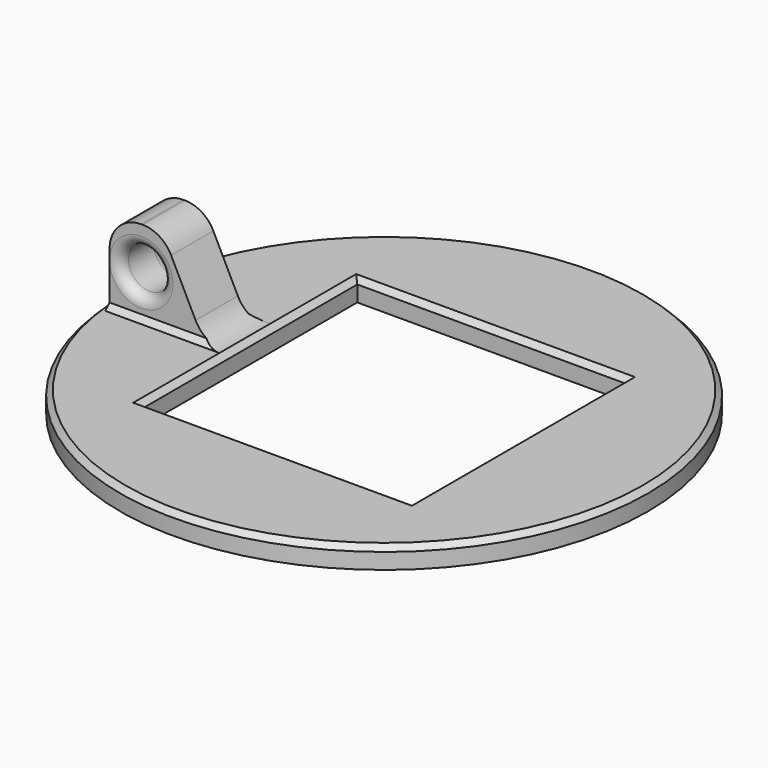
from build123d import *

# Parameters (mm, degrees)
F0_R          = 25
F0_W          = 25.4
F0_H          = 25.4
F1_DEPTH      = 2
F2_R          = 2
F3_DEPTH      = 2.5
F3_DEPTH_BACK = 2.5
F4_SIZE       = 0.5
F5_R          = 0.99999
F6_T4_DEPTH   = 5
F6_T9_DEPTH   = 5.1486606532
F6_T15_DEPTH  = 5.1486606532
F6_T18_DEPTH  = 20
F6_T20_DEPTH  = 14.2973213065


# Not quite as in the source:
# - a fillet or chamfer that OpenCascade refuses, or shapes differently, is made with other operations: its cross-section is extruded or revolved along the edge and cut away or added
# - a fillet or chamfer is up to 0.001 mm smaller than in the source, because OpenCascade refuses the exact size


with BuildPart() as f1:
    # F0 (on Top) → F1 (new body)
    with BuildSketch(Plane.XY):
        Circle(F0_R)
        Rectangle(F0_W, F0_H, mode=Mode.SUBTRACT)
    extrude(amount=F1_DEPTH)

    # F2 (on Front) → F3 (join, two sides)
    with BuildSketch(Plane.XZ) as f3_sk:
        Polygon((-24, 10), (-24, 1.4085747534), (-14.7320097312, 1.4085747534), (-19, 10), align=None)
        with Locations((-21, 6)):
            Circle(F2_R, mode=Mode.SUBTRACT)
    extrude(amount=F3_DEPTH)
    extrude(f3_sk.sketch, amount=-F3_DEPTH_BACK)

    # F4
    f4_edges = [f1.edges().sort_by_distance(p)[0] for p in [
        (0, 12.7, 2),
        (12.7, 0, 2),
        (0, -12.7, 2),
        (-12.7, 0, 2),
        (-25, 0, 2),
        (-19.512907, 2.5, 2),
        (-19.512907, -2.5, 2),
    ]]
    chamfer(f4_edges, length=F4_SIZE)

    # F5 (radius 1 in the source; OpenCascade refuses exactly that, so slightly less here)
    f5_edges = [f1.edges().sort_by_distance(p)[0] for p in [
        (-23, -2.5, 6),
        (-23, 2.5, 6),
    ]]
    fillet(f5_edges, radius=F5_R)

    # F6: fillet of radius 3 on 3 edges, made by hand


with BuildPart() as f6_tool2:
    # F6_s3 → F6_t4 (new body)
    with BuildSketch(Plane.XZ.offset(-2.5)):
        with BuildLine():
            ThreePointArc((-15.8530900959, 3.66529924), (-14.7468397832, 2.4500880133), (-13.1663497137, 2))
            Line((-13.1663497137, 2), (-15.025813975, 2))
            Line((-15.025813975, 2), (-15.8530900959, 3.66529924))
        make_face()
    extrude(amount=F6_T4_DEPTH)

    split(bisect_by=Plane(origin=(-5.6, 0, -5.6), x_dir=(0, 1, 0), z_dir=(-0.7071067812, 0, -0.7071067812)), keep=Keep.TOP)


with BuildPart() as f1_1:
    add(f1.part)

    # F6_t1: union F6_tool2
    add(f6_tool2.part)


with BuildPart() as f6_tool7:
    # F6_s8 → F6_t9 (new body)
    with BuildSketch(Plane.XZ.offset(-2.5)):
        with BuildLine():
            ThreePointArc((-15.8530900959, 3.66529924), (-14.7468397832, 2.4500880133), (-13.1663497137, 2))
            Line((-13.1663497137, 2), (-15.025813975, 2))
            Line((-15.025813975, 2), (-15.8530900959, 3.66529924))
        make_face()
    extrude(amount=-F6_T9_DEPTH)

    split(bisect_by=Plane(origin=(0, 2.5, 2.5), x_dir=(1, 0, 0), z_dir=(0, -0.7071067812, -0.7071067812)), keep=Keep.TOP)

    split(bisect_by=Plane(origin=(-5.6, 0, -5.6), x_dir=(0, 1, 0), z_dir=(-0.7071067812, 0, -0.7071067812)), keep=Keep.TOP)


with BuildPart() as f1_2:
    add(f1_1.part)

    # F6_t6: union F6_tool7
    add(f6_tool7.part)


with BuildPart() as f6_tool13:
    # F6_s14 → F6_t15 (new body)
    with BuildSketch(Plane.XZ.offset(2.5)):
        with BuildLine():
            ThreePointArc((-15.8530900959, 3.66529924), (-14.7468397832, 2.4500880133), (-13.1663497137, 2))
            Line((-13.1663497137, 2), (-15.025813975, 2))
            Line((-15.025813975, 2), (-15.8530900959, 3.66529924))
        make_face()
    extrude(amount=F6_T15_DEPTH)

    split(bisect_by=Plane(origin=(0, -2.5, 2.5), x_dir=(1, 0, 0), z_dir=(0, 0.7071067812, -0.7071067812)), keep=Keep.TOP)

    split(bisect_by=Plane(origin=(-5.6, 0, -5.6), x_dir=(0, 1, 0), z_dir=(-0.7071067812, 0, -0.7071067812)), keep=Keep.TOP)


with BuildPart() as f1_3:
    add(f1_2.part)

    # F6_t12: union F6_tool13
    add(f6_tool13.part)

    # F6_s19 → F6_t18 (cut)
    with BuildSketch(Plane.XZ.offset(-10)):
        with BuildLine():
            ThreePointArc((-24, 7), (-23.1213203436, 9.1213203436), (-21, 10))
            Line((-21, 10), (-24, 10))
            Line((-24, 10), (-24, 7))
        make_face()
    extrude(amount=F6_T18_DEPTH, mode=Mode.SUBTRACT)

    # F6_s21 → F6_t20 (cut)
    with BuildSketch(Plane.XZ.offset(-7.1486606532)):
        with BuildLine():
            ThreePointArc((-20.8594642613, 10), (-19.2789741917, 9.5499119867), (-18.1727238791, 8.33470076))
            Line((-18.1727238791, 8.33470076), (-19, 10))
            Line((-19, 10), (-20.8594642613, 10))
        make_face()
    extrude(amount=F6_T20_DEPTH, mode=Mode.SUBTRACT)


solid = f1_3.part
